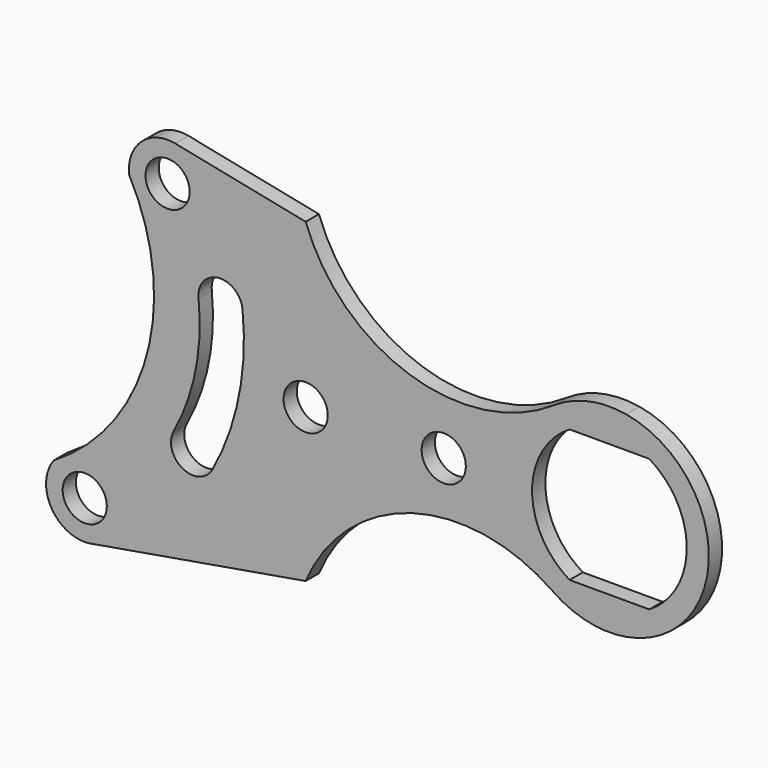
from build123d import *
from build123d import SkipClean  # not in build123d's __all__

# Parameters (mm, degrees)
F0_R     = 4
F1_DEPTH = 3
F3_DEPTH = 25


# Not quite as in the source:
# - a feature names something its author has since deleted; it is built from what else it names


with BuildPart() as f1:
    # F0 (on Front) → F1 (new body)
    with BuildSketch(Plane.XZ):
        with BuildLine():
            Line((47.076298262, 17.7403006666), (-34.5741482174, 34.3593566285))
            ThreePointArc((-34.5741482174, 34.3593566285), (-40.7303881594, 32.6323986455), (-42.9151879903, 26.6233784428))
            ThreePointArc((-42.9151879903, 26.6233784428), (-39.7469745445, -1.0840101596), (-56.5827821886, -23.3167009679))
            ThreePointArc((-56.5827821886, -23.3167009679), (-56.7807033092, -31.4037364957), (-49.2188462892, -34.2773465607))
            Line((-49.2188462892, -34.2773465607), (47.076298262, -17.7403006666))
            ThreePointArc((47.076298262, -17.7403006666), (62.0297047119, 0), (47.076298262, 17.7403006666))
        make_face()
        with Locations((-50.9702952881, -27.5)):
            Circle(F0_R, mode=Mode.SUBTRACT)
        with Locations((-10.9702952881, 0)):
            Circle(F0_R, mode=Mode.SUBTRACT)
        with Locations((-35.9702952881, 27.5)):
            Circle(F0_R, mode=Mode.SUBTRACT)
        with Locations((14.0297047119, 0)):
            Circle(F0_R, mode=Mode.SUBTRACT)
        with BuildLine():
            ThreePointArc((36.818602161, -12), (30.0297047119, 0), (36.818602161, 12))
            Line((36.818602161, 12), (51.2408072628, 12))
            ThreePointArc((51.2408072628, 12), (58.0297047119, 0), (51.2408072628, -12))
            Line((51.2408072628, -12), (36.818602161, -12))
        make_face(mode=Mode.SUBTRACT)
    extrude(amount=F1_DEPTH)

    # F2 (on face) → F3 (cut)
    with BuildSketch(Plane.XZ.offset(3)):
        with BuildLine():
            ThreePointArc((33.9762752, 14.9307921776), (40.2551488392, 17.5997934068), (47.076298262, 17.7403006666))
            Line((47.076298262, 17.7403006666), (-10.9702952881, 29.555050349))
            ThreePointArc((-10.9702952881, 29.555050349), (7.9384350476, 11.2875267012), (33.9762752, 14.9307921776))
        make_face()
        with BuildLine():
            ThreePointArc((47.076298262, -17.7403006666), (40.1280392566, -17.572051863), (33.7614970255, -14.7839071598))
            ThreePointArc((33.7614970255, -14.7839071598), (8.3202088026, -10.6027369585), (-10.9702952881, -27.7088113948))
            Line((-10.9702952881, -27.7088113948), (47.076298262, -17.7403006666))
        make_face()
        with BuildLine():
            ThreePointArc((-30.363862552, 11.08172749), (-30.8978419926, -0.5969747066), (-34.8691691907, -11.5926911146))
            ThreePointArc((-34.8691691907, -11.5926911146), (-33.2604899055, -17.0159881706), (-27.8371928496, -15.4073088854))
            ThreePointArc((-27.8371928496, -15.4073088854), (-23.0512344312, -2.1560609065), (-22.4077207465, 11.91827251))
            ThreePointArc((-22.4077207465, 11.91827251), (-26.8040641592, 15.4780709028), (-30.363862552, 11.08172749))
        make_face()
    with SkipClean():  # cleaning this boolean's faces spoils the solid; the shape is the same uncleaned
        extrude(amount=-F3_DEPTH, mode=Mode.SUBTRACT)


solid = f1.part
